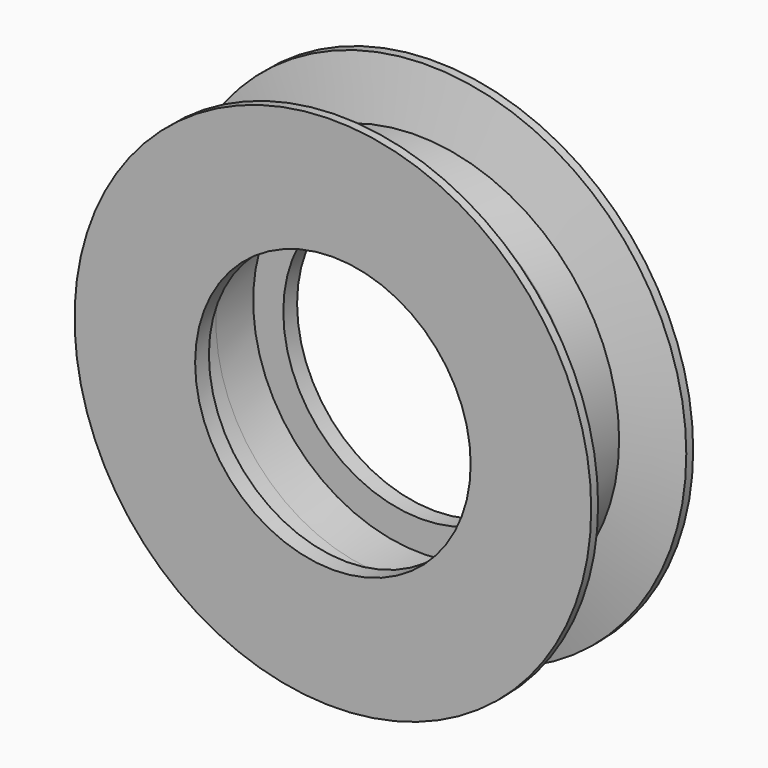
from build123d import *

# Parameters (mm, degrees)
F0_R        = 11.75
F0_R_2      = 9.75
F1_DEPTH    = 1.2
F2_R        = 15
F2_R_2      = 11.75
F2_R_3      = 9.75
F3_DEPTH    = 2.5
F4_S5_R     = 11.75
F4_T6_DEPTH = 23
F5_R        = 9.75
F5_R_2      = 8
F6_DEPTH    = 1


# Not quite as in the source:
# - a fillet or chamfer that OpenCascade refuses, or shapes differently, is made with other operations: its cross-section is extruded or revolved along the edge and cut away or added


with BuildPart() as f1:
    # F0 (on Front) → F1 (new body)
    with BuildSketch(Plane.XZ):
        Circle(F0_R)
        Circle(F0_R_2, mode=Mode.SUBTRACT)
    extrude(amount=F1_DEPTH)

    # F2 (on face) → F3 (join)
    with BuildSketch(Plane.XZ.offset(1.2)):
        Circle(F2_R)
        Circle(F2_R_2, mode=Mode.SUBTRACT)
        Circle(F2_R_2)
        Circle(F2_R_3, mode=Mode.SUBTRACT)
    extrude(amount=F3_DEPTH)

    # F4: chamfer of 2 x 8 on 1 edges, made by hand


with BuildPart() as f4_tool2:
    # F4_s3 → F4_t4 (revolve)
    with BuildSketch(Plane.XY):
        Polygon((7, -1.2), (15, -3.2), (15, -1.2), align=None)
    revolve(axis=Axis((0, -1.2, 0), (0, -1, 0)))

    # F4_s5 → F4_t6 (cut, symmetric)
    with BuildSketch(Plane.XZ.offset(2.2)):
        Circle(F4_S5_R)
    extrude(amount=F4_T6_DEPTH, both=True, mode=Mode.SUBTRACT)


with BuildPart() as f1_1:
    add(f1.part)

    # F4_t1: cut F4_tool2
    add(f4_tool2.part, mode=Mode.SUBTRACT)

    # F5 (on face) → F6 (join)
    with BuildSketch(Plane.XZ.offset(3.7)):
        Circle(F5_R)
        Circle(F5_R_2, mode=Mode.SUBTRACT)
    extrude(amount=-F6_DEPTH)


with BuildPart() as f7_1:
    # F7: instance of F1
    add(f1_1.part.mirror(Plane(origin=(0, 0, 0), x_dir=(1, 0, 0), z_dir=(0, 1, 0))))


solid = Compound([f1_1.part, f7_1.part])
